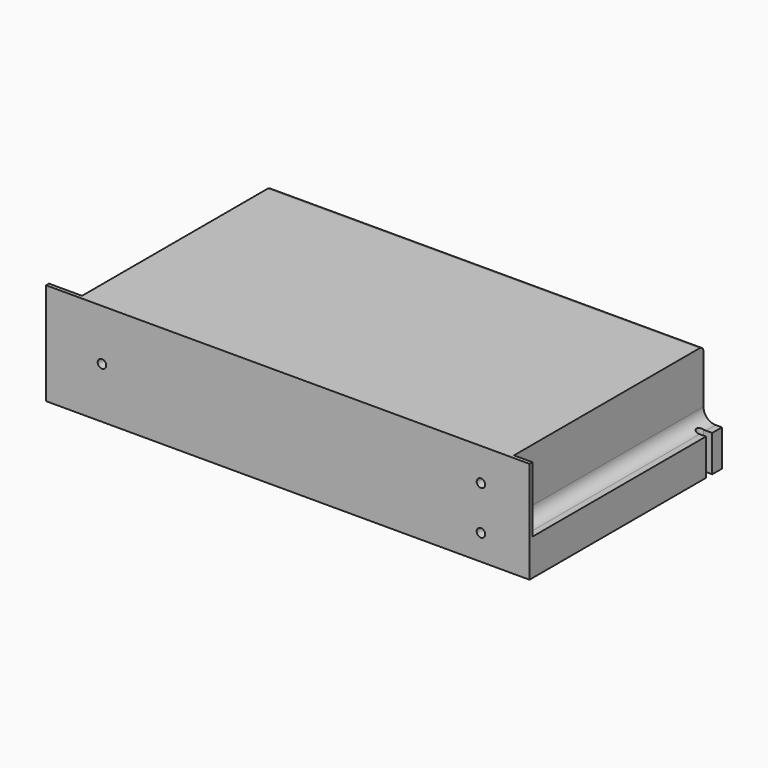
from build123d import *

# Parameters (mm, degrees)
F1_W      = 199
F1_H      = 42
F1_R      = 1.75
F2_DEPTH  = 99
F4_W      = 97.5
F4_H      = 27
F5_DEPTH  = 7.6
F6_R      = 5
F8_W      = 97.5
F8_H      = 40.5
F9_DEPTH  = 13.6
F10_W     = 68
F10_H     = 17.5
F11_DEPTH = 13.6
F12_R     = 2
F13_R     = 2
F15_R     = 1.6
F16_DEPTH = 42.001


# Not quite as in the source:
# - the program builds the solid bodies; features that only make, move or delete a surface that nothing else refers to are left out


with BuildPart() as f2:
    # F1 (on Front) → F2 (new body)
    with BuildSketch(Plane.XZ):
        Rectangle(F1_W, F1_H)
        with Locations((79.5, -10.5)):
            Circle(F1_R, mode=Mode.SUBTRACT)
        with Locations((-76.5, 0)):
            Circle(F1_R, mode=Mode.SUBTRACT)
        with Locations((79.5, 7.5)):
            Circle(F1_R, mode=Mode.SUBTRACT)
    extrude(amount=-F2_DEPTH)

    # F4 (on offset) → F5 (cut)
    with BuildSketch(Plane.YZ.offset(99.5)):
        with Locations((50.25, 7.5)):
            Rectangle(F4_W, F4_H)
    extrude(amount=-F5_DEPTH, mode=Mode.SUBTRACT)

    # F6
    f6_edges = [f2.edges().sort_by_distance(p)[0] for p in [
        (91.9, 50.25, -6),
    ]]
    fillet(f6_edges, radius=F6_R)

    # F8 (on offset) → F9 (cut)
    with BuildSketch(Plane(origin=(-99.5, 0, 0), x_dir=(0, -1, 0), z_dir=(-1, 0, 0))):
        with Locations((-50.25, 0.75)):
            Rectangle(F8_W, F8_H)
    extrude(amount=-F9_DEPTH, mode=Mode.SUBTRACT)

    # F10 (on offset) → F11 (join, through all)
    with BuildSketch(Plane(origin=(-99.5, 0, 0), x_dir=(0, -1, 0), z_dir=(-1, 0, 0))):
        with Locations((-52.6, -4.25)):
            Rectangle(F10_W, F10_H)
    extrude(amount=-F11_DEPTH)

    # F12
    f12_edges = [f2.edges().sort_by_distance(p)[0] for p in [
        (-99.5, 52.6, 4.5),
    ]]
    fillet(f12_edges, radius=F12_R)

    # F13
    f13_edges = [f2.edges().sort_by_distance(p)[0] for p in [
        (3, 99, 21),
    ]]
    fillet(f13_edges, radius=F13_R)

    # F15 (on face) → F16 (cut, through all)
    with BuildSketch(Plane(origin=(0, 0, -21), x_dir=(1, 0, 0), z_dir=(0, 0, -1))):
        with Locations((-96.3, -6.4)):
            Circle(F15_R)
        with BuildLine():
            Line((96, -94), (99.5, -94))
            Line((99.5, -94), (99.5, -90.8))
            Line((99.5, -90.8), (96, -90.8))
            ThreePointArc((96, -90.8), (97.1313708499, -91.2686291501), (97.6, -92.4))
            ThreePointArc((97.6, -92.4), (97.1313708499, -93.5313708499), (96, -94))
        make_face()
        with BuildLine():
            Line((96, -90.8), (96, -94))
            ThreePointArc((96, -94), (97.1313708499, -93.5313708499), (97.6, -92.4))
            ThreePointArc((97.6, -92.4), (97.1313708499, -91.2686291501), (96, -90.8))
        make_face()
        with BuildLine():
            ThreePointArc((96, -90.8), (94.4, -92.4), (96, -94))
            Line((96, -94), (96, -90.8))
        make_face()
    extrude(amount=-F16_DEPTH, mode=Mode.SUBTRACT)


solid = f2.part
